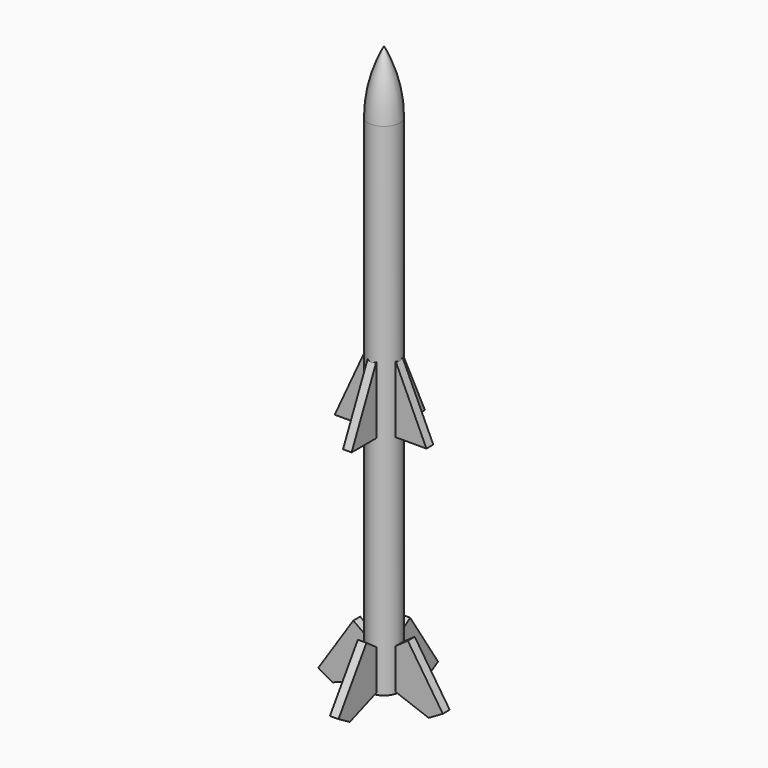
from build123d import *

# Parameters (mm, degrees)
F3_DEPTH = 0.2
F4_COUNT = 4


# Not quite as in the source:
# - a feature names something its author has since deleted; it is built from what else it names


with BuildPart() as f1:
    # F0 (on Front) → F1 (revolve)
    with BuildSketch(Plane.XZ):
        with BuildLine():
            Line((0, 26.25), (0, 0))
            Line((0, 0), (0.7291666667, 0))
            Line((0.7291666667, 0), (0.7291666667, 23.3333333333))
            ThreePointArc((0.7291666667, 23.3333333333), (0.5441123707, 24.836548926), (0, 26.25))
        make_face()
    revolve(axis=Axis((0, 0, 13.125), (0, 0, 1)))

    # F2 (on Front) → F3 (join, symmetric)
    with BuildSketch(Plane.XZ):
        Polygon((0, 15.1607510288), (0, 10.5208333333), (2.1354166667, 10.5208333333), align=None)
        Polygon((0, 1.4650106838), (0, 0.3376436782), (2.2395833333, -0.4861111111), (2.8993055556, -0.1041666667), (1.2708333333, 2.3611111111), align=None)
    extrude(amount=F3_DEPTH, both=True)

    # F4: F1 ×4 about axis
    f4_axis = Axis((0, 0, 0), (0, 0, 1))


with BuildPart() as f1_1:
    add(f1.part)
    for i in range(1, F4_COUNT):
        add(f1.part.rotate(f4_axis, i * 360 / F4_COUNT))


solid = f1_1.part
